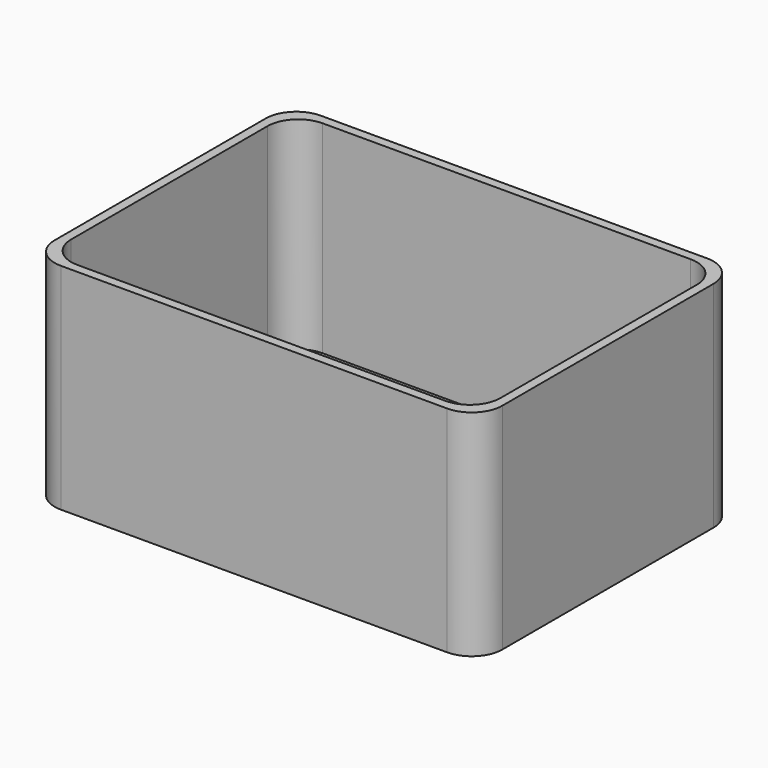
from build123d import *

# Parameters (mm, degrees)
F1_DEPTH = 2
F2_DEPTH = 35


with BuildPart() as f1:
    # F0 (on Top) → F1 (new body)
    with BuildSketch(Plane.XY):
        with BuildLine():
            Line((31.5, 26.5), (-31.5, 26.5))
            ThreePointArc((-31.5, 26.5), (-35.0355339059, 25.0355339059), (-36.5, 21.5))
            Line((-36.5, 21.5), (-36.5, -21.5))
            ThreePointArc((-36.5, -21.5), (-35.0355339059, -25.0355339059), (-31.5, -26.5))
            Line((-31.5, -26.5), (31.5, -26.5))
            ThreePointArc((31.5, -26.5), (35.0355339059, -25.0355339059), (36.5, -21.5))
            Line((36.5, -21.5), (36.5, 21.5))
            ThreePointArc((36.5, 21.5), (35.0355339059, 25.0355339059), (31.5, 26.5))
        make_face()
        with BuildLine():
            ThreePointArc((-35, 20), (-33.5355339059, 23.5355339059), (-30, 25))
            Line((-30, 25), (30, 25))
            ThreePointArc((30, 25), (33.5355339059, 23.5355339059), (35, 20))
            Line((35, 20), (35, -20))
            ThreePointArc((35, -20), (33.5355339059, -23.5355339059), (30, -25))
            Line((30, -25), (-30, -25))
            ThreePointArc((-30, -25), (-33.5355339059, -23.5355339059), (-35, -20))
            Line((-35, -20), (-35, 20))
        make_face(mode=Mode.SUBTRACT)
        with BuildLine():
            Line((30, 25), (-30, 25))
            ThreePointArc((-30, 25), (-33.5355339059, 23.5355339059), (-35, 20))
            Line((-35, 20), (-35, -20))
            ThreePointArc((-35, -20), (-33.5355339059, -23.5355339059), (-30, -25))
            Line((-30, -25), (30, -25))
            ThreePointArc((30, -25), (33.5355339059, -23.5355339059), (35, -20))
            Line((35, -20), (35, 20))
            ThreePointArc((35, 20), (33.5355339059, 23.5355339059), (30, 25))
        make_face()
    extrude(amount=F1_DEPTH)

    # F0 (on Top) → F2 (join)
    with BuildSketch(Plane.XY):
        with BuildLine():
            Line((31.5, 26.5), (-31.5, 26.5))
            ThreePointArc((-31.5, 26.5), (-35.0355339059, 25.0355339059), (-36.5, 21.5))
            Line((-36.5, 21.5), (-36.5, -21.5))
            ThreePointArc((-36.5, -21.5), (-35.0355339059, -25.0355339059), (-31.5, -26.5))
            Line((-31.5, -26.5), (31.5, -26.5))
            ThreePointArc((31.5, -26.5), (35.0355339059, -25.0355339059), (36.5, -21.5))
            Line((36.5, -21.5), (36.5, 21.5))
            ThreePointArc((36.5, 21.5), (35.0355339059, 25.0355339059), (31.5, 26.5))
        make_face()
        with BuildLine():
            ThreePointArc((-35, 20), (-33.5355339059, 23.5355339059), (-30, 25))
            Line((-30, 25), (30, 25))
            ThreePointArc((30, 25), (33.5355339059, 23.5355339059), (35, 20))
            Line((35, 20), (35, -20))
            ThreePointArc((35, -20), (33.5355339059, -23.5355339059), (30, -25))
            Line((30, -25), (-30, -25))
            ThreePointArc((-30, -25), (-33.5355339059, -23.5355339059), (-35, -20))
            Line((-35, -20), (-35, 20))
        make_face(mode=Mode.SUBTRACT)
    extrude(amount=F2_DEPTH)


solid = f1.part
